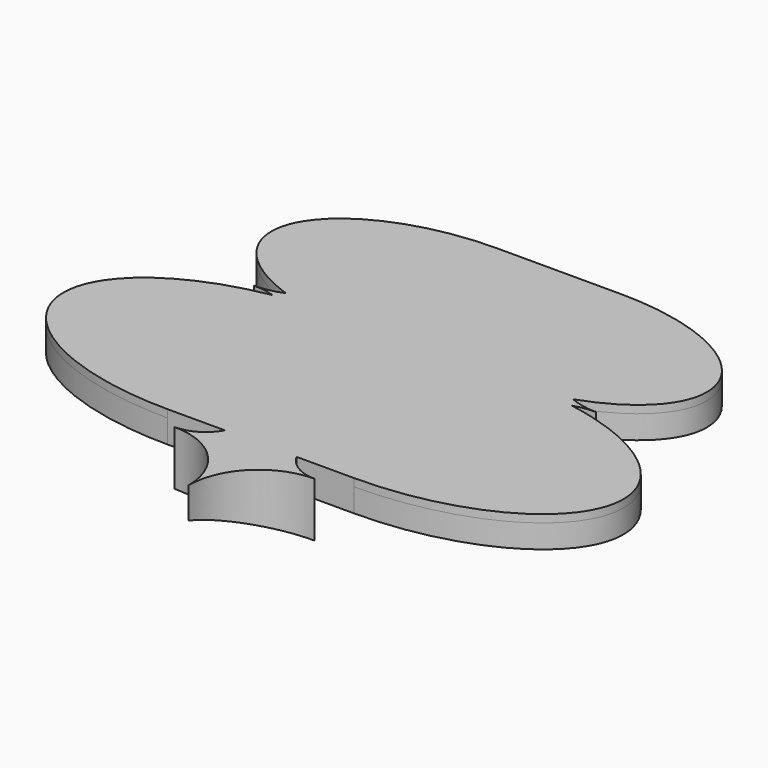
from build123d import *

# Parameters (mm, degrees)
F1_DEPTH       = 1.5875
F3_DEPTH       = 6.35
F5_DEPTH       = 11.1125
F6_W           = 3.175
F6_H           = 12.7
F7_DEPTH       = 4.7625
F8_W           = 3.175
F8_H           = 12.7
F9_DEPTH       = 4.7625
F11_DEPTH      = 57.1510001
F11_DEPTH_BACK = 57.1510001
F13_DEPTH      = 94.616


# Not quite as in the source:
# - ends of sketch curves that miss each other by under 0.0002 mm in the source are joined


with BuildPart() as f1:
    # F0 (on Top) → F1 (new body, symmetric)
    with BuildSketch(Plane.XY):
        with BuildLine():
            Line((12.7, 76.2), (-12.7, 76.2))
            add(Edge.make_bspline(
                [(-12.7, 76.2), (-38.5075450931, 76.2), (-43.7802754355, 61.9636280754), (-49.053005778, 47.7272561507), (-25.4, 41.91)],
                knots=[1.5707963268, 1.5707963268, 1.5707963268, 2.9358342306, 2.9358342306, 4.3008721343, 4.3008721343, 4.3008721343], degree=2, weights=[1, 0.7759863542, 1, 0.7759863542, 1]))
            add(Edge.make_bspline(
                [(-25.4, 41.91), (-59.9465199005, 38.6756961659), (-57.0165429182, 19.337848083), (-54.086565936, 0), (-19.05, 0)],
                knots=[1.738244406, 1.738244406, 1.738244406, 3.2253166932, 3.2253166932, 4.7123889804, 4.7123889804, 4.7123889804], degree=2, weights=[1, 0.7360795678, 1, 0.7360795678, 1]))
            Line((-19.05, 0), (19.05, 0))
            add(Edge.make_bspline(
                [(19.05, 0), (54.086565936, 0), (57.0165429182, 19.337848083), (59.9465199005, 38.6756961659), (25.4, 41.91)],
                knots=[1.5707963268, 1.5707963268, 1.5707963268, 3.057868614, 3.057868614, 4.5449409012, 4.5449409012, 4.5449409012], degree=2, weights=[1, 0.7360795678, 1, 0.7360795678, 1]))
            add(Edge.make_bspline(
                [(25.4, 41.91), (49.053005778, 47.7272561507), (43.7802754355, 61.9636280754), (38.5075450931, 76.2), (12.7, 76.2)],
                knots=[1.9823131729, 1.9823131729, 1.9823131729, 3.3473510766, 3.3473510766, 4.7123889804, 4.7123889804, 4.7123889804], degree=2, weights=[1, 0.7759863542, 1, 0.7759863542, 1]))
        make_face()
    extrude(amount=F1_DEPTH, both=True)

    # F2 (on Top) → F3 (join, symmetric)
    with BuildSketch(Plane.XY):
        with BuildLine():
            Line((0, 12.7), (-19.05, 12.7))
            add(Edge.make_bspline(
                [(-20.32, 41.148), (-40.7772217963, 40.3172874256), (-40.1607644877, 26.5086437128), (-39.5443071791, 12.7), (-19.05, 12.7)],
                knots=[1.6309642847, 1.6309642847, 1.6309642847, 3.1716766325, 3.1716766325, 4.7123889804, 4.7123889804, 4.7123889804], degree=2, weights=[1, 0.7176626789, 1, 0.7176626789, 1]))
            add(Edge.make_bspline(
                [(-12.7, 63.5), (-28.1845270559, 63.5), (-31.3481652613, 54.2199945973), (-34.5118034668, 44.9399891945), (-20.32, 41.148)],
                knots=[4.7123889804, 4.7123889804, 4.7123889804, 6.0774268841, 6.0774268841, 7.4424647879, 7.4424647879, 7.4424647879], degree=2, weights=[1, 0.7759863542, 1, 0.7759863542, 1]))
            Line((-12.7, 63.5), (0, 63.5))
            Line((0, 63.5), (6.35, 63.5))
            Line((6.35, 63.5), (6.35, 76.2))
            Line((6.35, 76.2), (-12.7, 76.2))
            add(Edge.make_bspline(
                [(-12.7, 76.2), (-38.5075450931, 76.2), (-43.7802754355, 61.9636280754), (-49.053005778, 47.7272561507), (-25.4, 41.91)],
                knots=[1.5707963268, 1.5707963268, 1.5707963268, 2.9358342306, 2.9358342306, 4.3008721343, 4.3008721343, 4.3008721343], degree=2, weights=[1, 0.7759863542, 1, 0.7759863542, 1]))
            add(Edge.make_bspline(
                [(-25.4, 41.91), (-59.9465199005, 38.6756961659), (-57.0165429182, 19.337848083), (-54.086565936, 0), (-19.05, 0)],
                knots=[1.738244406, 1.738244406, 1.738244406, 3.2253166932, 3.2253166932, 4.7123889804, 4.7123889804, 4.7123889804], degree=2, weights=[1, 0.7360795678, 1, 0.7360795678, 1]))
            Line((-19.05, 0), (19.05, 0))
            add(Edge.make_bspline(
                [(19.05, 0), (54.086565936, 0), (57.0165429182, 19.337848083), (59.9465199005, 38.6756961659), (25.4, 41.91)],
                knots=[1.5707963268, 1.5707963268, 1.5707963268, 3.057868614, 3.057868614, 4.5449409012, 4.5449409012, 4.5449409012], degree=2, weights=[1, 0.7360795678, 1, 0.7360795678, 1]))
            add(Edge.make_bspline(
                [(25.4, 41.91), (49.053005778, 47.7272561507), (43.7802754355, 61.9636280754), (38.5075450931, 76.2), (12.7, 76.2)],
                knots=[1.9823131729, 1.9823131729, 1.9823131729, 3.3473510766, 3.3473510766, 4.7123889804, 4.7123889804, 4.7123889804], degree=2, weights=[1, 0.7759863542, 1, 0.7759863542, 1]))
            Line((12.7, 76.2), (9.525, 76.2))
            Line((9.525, 76.2), (9.525, 63.5))
            Line((9.525, 63.5), (12.7, 63.5))
            add(Edge.make_bspline(
                [(20.32, 41.148), (34.5118034668, 44.9399891945), (31.3481652613, 54.2199945973), (28.1845270559, 63.5), (12.7, 63.5)],
                knots=[5.1239058265, 5.1239058265, 5.1239058265, 6.4889437302, 6.4889437302, 7.853981634, 7.853981634, 7.853981634], degree=2, weights=[1, 0.7759863542, 1, 0.7759863542, 1]))
            add(Edge.make_bspline(
                [(19.05, 12.7), (39.5443071791, 12.7), (40.1607644877, 26.5086437128), (40.7772217963, 40.3172874256), (20.32, 41.148)],
                knots=[4.7123889804, 4.7123889804, 4.7123889804, 6.2531013282, 6.2531013282, 7.7938136761, 7.7938136761, 7.7938136761], degree=2, weights=[1, 0.7176626789, 1, 0.7176626789, 1]))
            Line((19.05, 12.7), (0, 12.7))
        make_face()
    extrude(amount=F3_DEPTH, both=True)

    # F4 (on Top) → F5 (join, symmetric)
    with BuildSketch(Plane.XY):
        with BuildLine():
            Line((6.35, 48.26), (6.35, 76.2))
            Line((6.35, 76.2), (-6.35, 76.2))
            Line((-6.35, 76.2), (-6.35, 48.26))
            Line((-6.35, 48.26), (-12.7, 48.26))
            ThreePointArc((-12.7, 48.26), (-18.3126600757, 50.5848399243), (-20.6375, 56.1975))
            ThreePointArc((-20.6375, 56.1975), (-24.8222118638, 46.0947118638), (-34.925, 41.91))
            ThreePointArc((-34.925, 41.91), (-24.8222118638, 37.7252881362), (-20.6375, 27.6225))
            ThreePointArc((-20.6375, 27.6225), (-18.3126600757, 33.2351600757), (-12.7, 35.56))
            Line((-12.7, 35.56), (-6.35, 35.56))
            Line((-6.35, 35.56), (-6.3499892508, 3.8099982085))
            ThreePointArc((-6.3499892508, 3.8099982085), (-8.674852257, -1.8026576282), (-14.2875129886, -4.1274959691))
            ThreePointArc((-14.2875129886, -4.1274959691), (-4.184726033, -8.3122106832), (-1.70195e-05, -18.415))
            ThreePointArc((-1.70195e-05, -18.415), (4.1846976946, -8.3122130444), (14.2874870114, -4.1275040309))
            ThreePointArc((14.2874870114, -4.1275040309), (8.6748275917, -1.8026625231), (6.3499892508, 3.8099982085))
            Line((6.3499892508, 3.8099982085), (6.35, 35.56))
            Line((6.35, 35.56), (12.7, 35.56))
            ThreePointArc((12.7, 35.56), (18.3126600757, 33.2351600757), (20.6375, 27.6225))
            ThreePointArc((20.6375, 27.6225), (24.8222118638, 37.7252881362), (34.925, 41.91))
            ThreePointArc((34.925, 41.91), (24.8222118638, 46.0947118638), (20.6375, 56.1975))
            ThreePointArc((20.6375, 56.1975), (18.3126600757, 50.5848399243), (12.7, 48.26))
            Line((12.7, 48.26), (6.35, 48.26))
        make_face()
    extrude(amount=F5_DEPTH, both=True)

    # F6 (on face) → F7 (join, through all)
    with BuildSketch(Plane(origin=(0, 0, -6.35), x_dir=(1, 0, 0), z_dir=(0, 0, -1))):
        with Locations((7.9375, -69.85)):
            Rectangle(F6_W, F6_H)
    extrude(amount=-F7_DEPTH)

    # F8 (on face) → F9 (cut, through all)
    with BuildSketch(Plane(origin=(0, 0, -6.35), x_dir=(1, 0, 0), z_dir=(0, 0, -1))):
        with Locations((-7.9375, -69.85)):
            Rectangle(F8_W, F8_H)
    extrude(amount=-F9_DEPTH, mode=Mode.SUBTRACT)

    # F10 (on Right) → F11 (cut, two sides)
    with BuildSketch(Plane.YZ) as f11_sk:
        Polygon((-18.415, 6.35), (-4.1275040309, 11.1125), (-18.415, 11.1125), align=None)
        Polygon((-4.1275040309, 11.1125), (63.5, 6.35), (76.2, 6.35), (76.2, 11.1125), align=None)
        Polygon((-4.1275040309, -11.1125), (-18.415, -6.35), (-18.415, -11.1125), align=None)
        Polygon((63.5, -6.35), (-4.1275040309, -11.1125), (76.2, -11.1125), (76.2, -6.35), align=None)
    extrude(amount=-F11_DEPTH, mode=Mode.SUBTRACT)
    extrude(f11_sk.sketch, amount=F11_DEPTH_BACK, mode=Mode.SUBTRACT)

    # F12 (on face) → F13 (cut, through all)
    with BuildSketch(Plane(origin=(0, 76.2, 0), x_dir=(-1, 0, 0), z_dir=(0, 1, 0))):
        Polygon((-57.15, 0), (-12.7, 0), (12.7, 0), (57.15, 0), (57.15, 6.35), (57.15, 11.1125), (-57.15, 11.1125), align=None)
    extrude(amount=-F13_DEPTH, mode=Mode.SUBTRACT)


solid = f1.part
